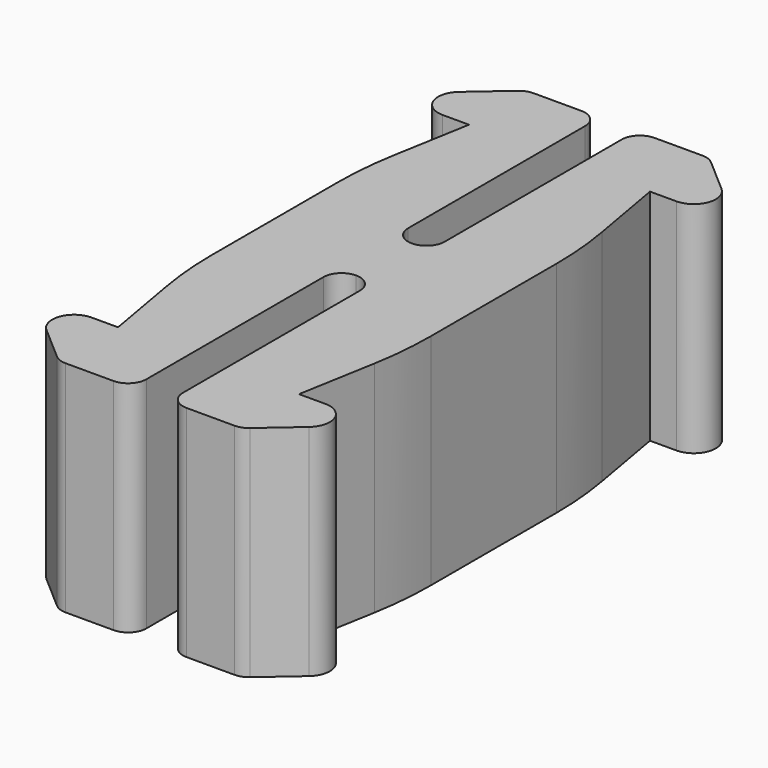
from build123d import *

# Parameters (mm, degrees)
F1_DEPTH = 3
F2_R     = 0.24999
F3_R     = 5


# Not quite as in the source:
# - a fillet or chamfer is up to 0.001 mm smaller than in the source, because OpenCascade refuses the exact size


with BuildPart() as f1:
    # F0 (on Top) → F1 (new body)
    with BuildSketch(Plane.XY):
        with BuildLine():
            Line((-1.5, 1.5121936516), (-1.5, 0))
            Line((-1.5, 0), (-1.5, -1.5121936516))
            Line((-1.5, -1.5121936516), (-1.2376595987, -3))
            Line((-1.2376595987, -3), (-1.5982141028, -3))
            ThreePointArc((-1.5982141028, -3), (-1.8792268389, -3.1949674233), (-1.7949840479, -3.5264543855))
            Line((-1.7949840479, -3.5264543855), (-1.25, -4))
            Line((-1.25, -4), (-0.25, -4))
            Line((-0.25, -4), (-0.25, -0.4752505826))
            Line((-0.25, -0.4752505826), (0, -0.4752505826))
            Line((0, -0.4752505826), (0.25, -0.4752505826))
            Line((0.25, -0.4752505826), (0.25, -4))
            Line((0.25, -4), (1.25, -4))
            Line((1.25, -4), (1.7949840479, -3.5264543855))
            ThreePointArc((1.7949840479, -3.5264543855), (1.8792268389, -3.1949674233), (1.5982141028, -3))
            Line((1.5982141028, -3), (1.2376595987, -3))
            Line((1.2376595987, -3), (1.5, -1.5121936516))
            Line((1.5, -1.5121936516), (1.5, 1.5121936516))
            Line((1.5, 1.5121936516), (1.2376595987, 3))
            Line((1.2376595987, 3), (1.5982141028, 3))
            ThreePointArc((1.5982141028, 3), (1.8792268389, 3.1949674233), (1.7949840479, 3.5264543855))
            Line((1.7949840479, 3.5264543855), (1.25, 4))
            Line((1.25, 4), (0.25, 4))
            Line((0.25, 4), (0.25, 0.4752505826))
            Line((0.25, 0.4752505826), (0, 0.4752505826))
            Line((0, 0.4752505826), (-0.25, 0.4752505826))
            Line((-0.25, 0.4752505826), (-0.25, 4))
            Line((-0.25, 4), (-1.25, 4))
            Line((-1.25, 4), (-1.7949840479, 3.5264543855))
            ThreePointArc((-1.7949840479, 3.5264543855), (-1.8792268389, 3.1949674233), (-1.5982141028, 3))
            Line((-1.5982141028, 3), (-1.2376595987, 3))
            Line((-1.2376595987, 3), (-1.5, 1.5121936516))
        make_face()
    extrude(amount=F1_DEPTH)

    # F2 (radius 0.25 in the source; OpenCascade refuses exactly that, so slightly less here)
    f2_edges = [f1.edges().sort_by_distance(p)[0] for p in [
        (-1.25, 4, 1.5),
        (-0.25, 4, 1.5),
        (0.25, 4, 1.5),
        (1.25, 4, 1.5),
        (-0.25, 0.475251, 1.5),
        (0.25, 0.475251, 1.5),
        (-0.25, -0.475251, 1.5),
        (0.25, -0.475251, 1.5),
        (-1.25, -4, 1.5),
        (-0.25, -4, 1.5),
        (0.25, -4, 1.5),
        (1.25, -4, 1.5),
    ]]
    fillet(f2_edges, radius=F2_R)

    # F3
    f3_edges = [f1.edges().sort_by_distance(p)[0] for p in [
        (-1.5, -1.512194, 1.5),
        (-1.5, 1.512194, 1.5),
        (1.5, -1.512194, 1.5),
        (1.5, 1.512194, 1.5),
    ]]
    fillet(f3_edges, radius=F3_R)


solid = f1.part
